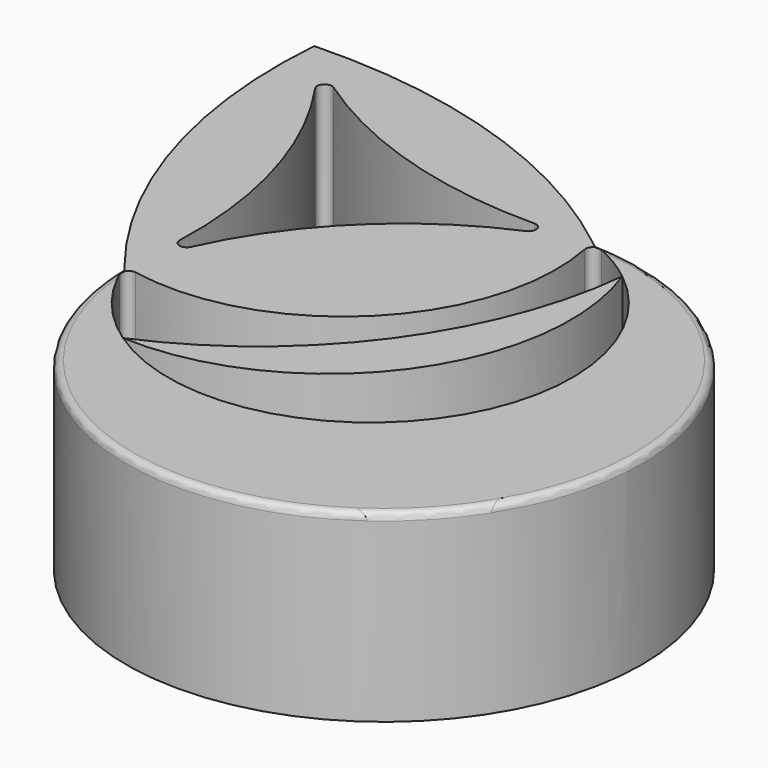
from build123d import *

# Parameters (mm, degrees)
F1_DEPTH     = 25
F2_T3_ANGLE  = 277.2561785364
F2_S4_R      = 74.3476887017
F2_T5_DEPTH  = 55
F2_T8_ANGLE  = 277.2561785364
F2_S9_R      = 27.4134694575
F2_T10_DEPTH = 55
F2_T13_ANGLE = 277.2561785364
F2_S14_R     = 77.8887101347
F2_T15_DEPTH = 55


# Not quite as in the source:
# - a fillet or chamfer that OpenCascade refuses, or shapes differently, is made with other operations: its cross-section is extruded or revolved along the edge and cut away or added


with BuildPart() as f1:
    # F0 (on Top) → F1 (new body)
    with BuildSketch(Plane.XY):
        with BuildLine():
            ThreePointArc((-51.1308461428, 51.9806705415), (-48.1352657569, 24.4924590263), (-35.3019214927, 0))
            ThreePointArc((-35.3019214927, 0), (-11.9360610306, 11.9222525038), (0, 35.2810621262))
            ThreePointArc((0, 35.2810621262), (-24.0781203636, 48.1846884371), (-51.1308461428, 51.9806705415))
        make_face()
        with BuildLine():
            ThreePointArc((-44.9915609391, 44.4670594009), (-44.8752915408, 45.7424555435), (-43.5997894412, 45.8575567498))
            ThreePointArc((-43.5997894412, 45.8575567498), (-26.3906174951, 37.5147808031), (-7.4646334829, 34.7643919688))
            ThreePointArc((-7.4646334829, 34.7643919688), (-6.477046058, 33.9713642367), (-7.0589584771, 32.8463754179))
            ThreePointArc((-7.0589584771, 32.8463754179), (-22.1189253759, 22.7184704393), (-32.5153694664, 7.8426171017))
            ThreePointArc((-32.5153694664, 7.8426171017), (-33.6547664634, 7.2819452695), (-34.4255319223, 8.2911523976))
            ThreePointArc((-34.4255319223, 8.2911523976), (-36.7907949795, 27.2313042006), (-44.9915609391, 44.4670594009))
        make_face(mode=Mode.SUBTRACT)
        with BuildLine():
            ThreePointArc((0, 35.2810621262), (-11.9360610306, 11.9222525038), (-35.3019214927, 0))
            ThreePointArc((-35.3019214927, 0), (24.438361689, -24.4736760144), (0, 35.2810621262))
        make_face()
        with BuildLine():
            ThreePointArc((-25.0962880995, -13.0191033564), (-30.5834095399, -8.0614766695), (-34.5457372408, -1.817557767))
            ThreePointArc((-34.5457372408, -1.817557767), (-34.4238128575, -0.7835364223), (-33.4487624549, -0.4183756234))
            ThreePointArc((-33.4487624549, -0.4183756234), (-7.550944031, 7.5345428735), (0.4172802234, 33.4276561272))
            ThreePointArc((0.4172802234, 33.4276561272), (0.7830172712, 34.4024905278), (1.8171104998, 34.5238037218))
            ThreePointArc((1.8171104998, 34.5238037218), (4.7089665972, 32.9790968837), (7.3957298922, 31.1001998934))
            ThreePointArc((7.3957298922, 31.1001998934), (12.4436027104, -6.6415033518), (-25.0962880995, -13.0191033564))
        make_face(mode=Mode.SUBTRACT)
    extrude(amount=F1_DEPTH)

    # F2: fillet of radius 1 on 1 edges, made by hand


with BuildPart() as f1b:
    # F0 (on Top) → F1, piece 2 (new body)
    with BuildSketch(Plane.XY):
        with BuildLine():
            ThreePointArc((7.3957298922, 31.1001998934), (-2.8774572569, 4.6418152739), (-25.0962880995, -13.0191033564))
            ThreePointArc((-25.0962880995, -13.0191033564), (2.9683883517, 0.3365949576), (7.3957298922, 31.1001998934))
        make_face()
    extrude(amount=F1_DEPTH)


with BuildPart() as f2_tool1:
    # F2_s2 → F2_t3 (revolve)
    with BuildSketch(Plane(origin=(0.0166906563, 0.2620049283, 0), x_dir=(0, 0, 1), z_dir=(0.0635747294, 0.9979770808, 0))):
        with BuildLine():
            ThreePointArc((24, -35.320399384), (24.7071067812, -35.0275061652), (25, -34.320399384))
            Line((25, -34.320399384), (25, -35.320399384))
            Line((25, -35.320399384), (24, -35.320399384))
        make_face()
    revolve(axis=Axis((-0.3030605857, 0.2823742324, 25), (0, 0, 1)), revolution_arc=F2_T3_ANGLE)

    # F2_s4 → F2_t5 (cut, symmetric)
    with BuildSketch(Plane.XY.offset(24.5)):
        with Locations((22.9879016294, 46.1505724307)):
            Circle(F2_S4_R)
    extrude(amount=F2_T5_DEPTH, both=True, mode=Mode.SUBTRACT)


with BuildPart() as f2_tool6:
    # F2_s7 → F2_t8 (revolve)
    with BuildSketch(Plane(origin=(0.0166906563, 0.2620049283, 0), x_dir=(0, 0, 1), z_dir=(0.0635747294, 0.9979770808, 0))):
        with BuildLine():
            ThreePointArc((24, -35.320399384), (24.7071067812, -35.0275061652), (25, -34.320399384))
            Line((25, -34.320399384), (25, -35.320399384))
            Line((25, -35.320399384), (24, -35.320399384))
        make_face()
    revolve(axis=Axis((-0.3030605857, 0.2823742324, 25), (0, 0, 1)), revolution_arc=F2_T8_ANGLE)

    # F2_s9 → F2_t10 (cut, symmetric)
    with BuildSketch(Plane.XY.offset(24.5)):
        with Locations((-9.6298182077, 9.6146461515)):
            Circle(F2_S9_R)
    extrude(amount=F2_T10_DEPTH, both=True, mode=Mode.SUBTRACT)


with BuildPart() as f2_tool11:
    # F2_s12 → F2_t13 (revolve)
    with BuildSketch(Plane(origin=(0.0166906563, 0.2620049283, 0), x_dir=(0, 0, 1), z_dir=(0.0635747294, 0.9979770808, 0))):
        with BuildLine():
            ThreePointArc((24, -35.320399384), (24.7071067812, -35.0275061652), (25, -34.320399384))
            Line((25, -34.320399384), (25, -35.320399384))
            Line((25, -35.320399384), (24, -35.320399384))
        make_face()
    revolve(axis=Axis((-0.3030605857, 0.2823742324, 25), (0, 0, 1)), revolution_arc=F2_T13_ANGLE)

    # F2_s14 → F2_t15 (cut, symmetric)
    with BuildSketch(Plane.XY.offset(24.5)):
        with Locations((-48.2599157967, -25.8551112391)):
            Circle(F2_S14_R)
    extrude(amount=F2_T15_DEPTH, both=True, mode=Mode.SUBTRACT)


with BuildPart() as f1_1:
    add(f1.part)

    # F2_t16: cut F2_tool1, F2_tool6, F2_tool11
    add([f2_tool1.part, f2_tool6.part, f2_tool11.part], mode=Mode.SUBTRACT)


solid = Compound([f1b.part, f1_1.part])
